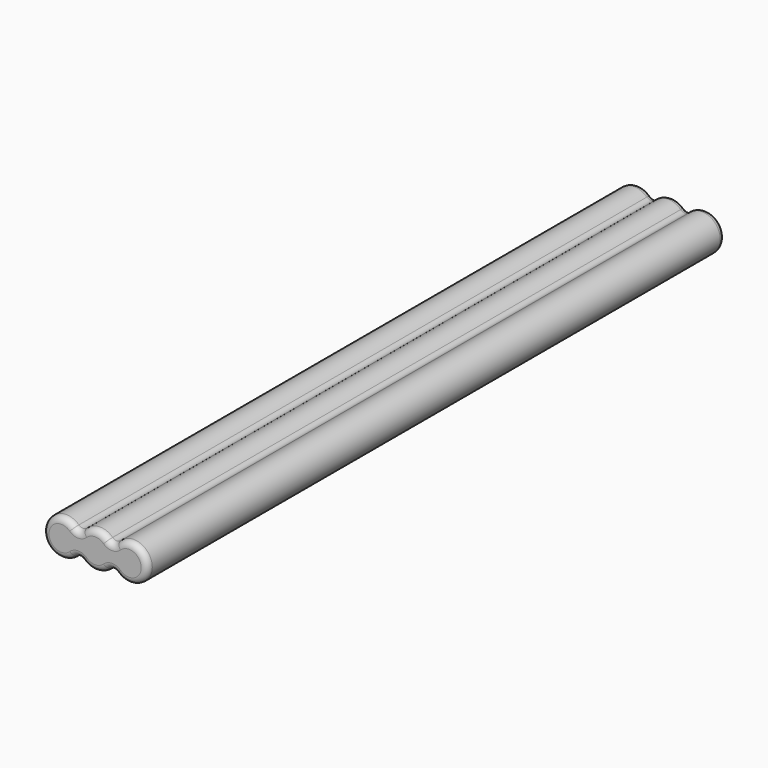
from build123d import *

# Parameters (mm, degrees)
F1_DEPTH = 74.6125
F2_R     = 1.27


with BuildPart() as f1:
    # F0 (on Front) → F1 (new body, symmetric)
    with BuildSketch(Plane.XZ):
        with BuildLine():
            ThreePointArc((3.4925, -1.5226765087), (10.795, 0), (3.4925, 1.5226765087))
            ThreePointArc((3.4925, 1.5226765087), (0, 3.81), (-3.4925, 1.5226765087))
            ThreePointArc((-3.4925, 1.5226765087), (-10.795, 0), (-3.4925, -1.5226765087))
            ThreePointArc((-3.4925, -1.5226765087), (0, -3.81), (3.4925, -1.5226765087))
        make_face()
    extrude(amount=F1_DEPTH, both=True)

    # F2
    f2_edges = [f1.edges().sort_by_distance(p)[0] for p in [
        (3.4925, 0, -1.522677),
        (10.795, 74.6125, 0),
        (3.4925, 0, 1.522677),
        (10.795, -74.6125, 0),
        (0, 74.6125, 3.81),
        (-3.4925, 0, 1.522677),
        (0, -74.6125, 3.81),
        (-10.795, 74.6125, 0),
        (-3.4925, 0, -1.522677),
        (-10.795, -74.6125, 0),
        (0, 74.6125, -3.81),
        (0, -74.6125, -3.81),
    ]]
    fillet(f2_edges, radius=F2_R)


solid = f1.part
